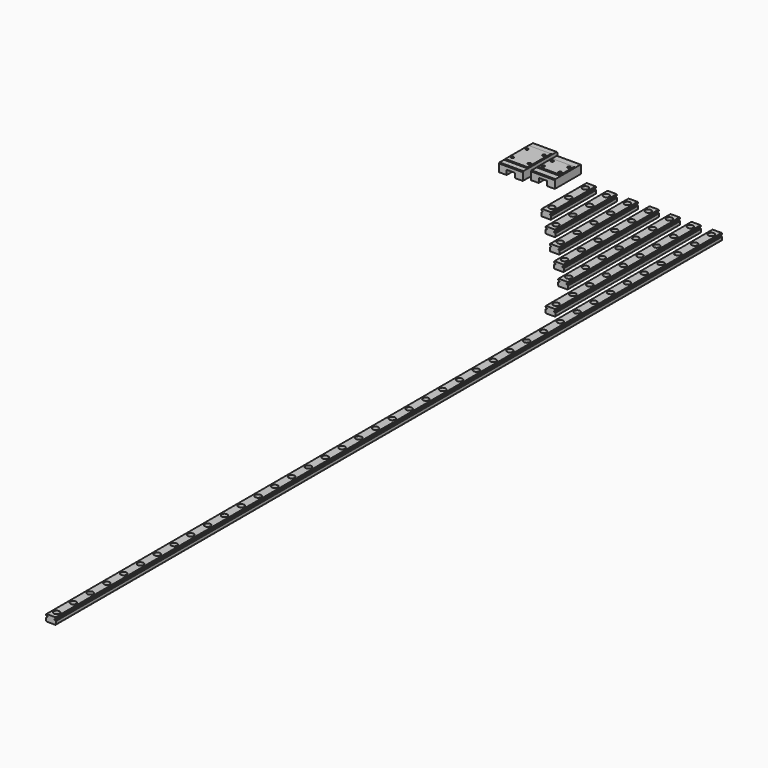
from build123d import *

# Parameters (mm, degrees)
F1_DEPTH         = 40
F2_DEPTH         = 55
F3_DEPTH         = 70
F4_DEPTH         = 85
F5_DEPTH         = 100
F6_DEPTH         = 130
F7_DEPTH         = 595
F9_D             = 2.4
F9_CBORE_D       = 4.2
F9_CBORE_DEPTH   = 2.3
F9_2_D           = 2.4
F9_2_CBORE_D     = 4.2
F9_2_CBORE_DEPTH = 2.3
F9_3_D           = 2.4
F9_3_CBORE_D     = 4.2
F9_3_CBORE_DEPTH = 2.3
F9_4_D           = 2.4
F9_4_CBORE_D     = 4.2
F9_4_CBORE_DEPTH = 2.3
F9_5_D           = 2.4
F9_5_CBORE_D     = 4.2
F9_5_CBORE_DEPTH = 2.3
F9_6_D           = 2.4
F9_6_CBORE_D     = 4.2
F9_6_CBORE_DEPTH = 2.3
F9_7_D           = 2.4
F9_7_CBORE_D     = 4.2
F9_7_CBORE_DEPTH = 2.3
F11_DEPTH        = 6.75
F13_DEPTH        = 5
F14_DEPTH        = 10.9
F16_DEPTH        = 4.5
F18_D            = 2
F18_DEPTH        = 2.5
F18_TIP          = 0.600860619
F18_2_D          = 2
F18_2_DEPTH      = 2.5
F18_2_TIP        = 0.600860619
F19_SIZE         = 0.49999
F19_2_SIZE       = 0.49999


# Not quite as in the source:
# - a fillet or chamfer is up to 0.001 mm smaller than in the source, because OpenCascade refuses the exact size


with BuildPart() as f1:
    # F0 (on Front) → F1 (new body)
    with BuildSketch(Plane.XZ):
        with BuildLine():
            Line((-3.2171572875, -2.4), (3.2171572875, -2.4))
            Line((3.2171572875, -2.4), (3.5, -2.1171572875))
            Line((3.5, -2.1171572875), (3.5, 0.1030976998))
            ThreePointArc((3.5, 0.1030976998), (3.2252249424, 0.2606627579), (3.036437636, 0.515))
            Line((3.036437636, 0.515), (2.6, 0.515))
            Line((2.6, 0.515), (2.6, 1.165))
            Line((2.6, 1.165), (3.036437636, 1.165))
            ThreePointArc((3.036437636, 1.165), (3.2252249424, 1.4193372421), (3.5, 1.5769023002))
            Line((3.5, 1.5769023002), (3.5, 2.1171572875))
            Line((3.5, 2.1171572875), (3.2171572875, 2.4))
            Line((3.2171572875, 2.4), (-3.2171572875, 2.4))
            Line((-3.2171572875, 2.4), (-3.5, 2.1171572875))
            Line((-3.5, 2.1171572875), (-3.5, 1.5769023002))
            ThreePointArc((-3.5, 1.5769023002), (-3.2252249424, 1.4193372421), (-3.036437636, 1.165))
            Line((-3.036437636, 1.165), (-2.6, 1.165))
            Line((-2.6, 1.165), (-2.6, 0.515))
            Line((-2.6, 0.515), (-3.036437636, 0.515))
            ThreePointArc((-3.036437636, 0.515), (-3.2252249424, 0.2606627579), (-3.5, 0.1030976998))
            Line((-3.5, 0.1030976998), (-3.5, -2.1171572875))
            Line((-3.5, -2.1171572875), (-3.2171572875, -2.4))
        make_face()
    extrude(amount=F1_DEPTH)

    # F9 (through all)
    with Locations(Plane.XY.offset(2.4)):
        with Locations((0, -5), (0, -20), (0, -35), (15, -5), (15, -20), (15, -35), (15, -50), (30, -5), (45, -5), (60, -5), (75, -5), (90, -5), (60, -20), (45, -20), (30, -20), (60, -35), (90, -65), (90, -50), (45, -50), (45, -35), (75, -50), (75, -65), (30, -50), (30, -35), (60, -65), (60, -50), (45, -65), (30, -65), (90, -35), (90, -20), (75, -20), (75, -35), (90, -95), (75, -95), (60, -95), (90, -110), (75, -110), (90, -125), (75, -125), (90, -80), (75, -80), (60, -80), (45, -80), (90, -305), (90, -290), (90, -215), (90, -200), (90, -185), (90, -350), (90, -320), (90, -335), (90, -245), (90, -230), (90, -140), (90, -365), (90, -380), (90, -260), (90, -275), (90, -395), (90, -155), (90, -170), (90, -530), (90, -545), (90, -455), (90, -440), (90, -425), (90, -560), (90, -575), (90, -590), (90, -470), (90, -485), (90, -500), (90, -515), (90, -410), (90, -410), (90, -425), (90, -440), (90, -455), (90, -470), (90, -485), (90, -500), (90, -515), (90, -530), (90, -545), (90, -560), (90, -575), (90, -590)):
            CounterBoreHole(F9_D / 2, F9_CBORE_D / 2, F9_CBORE_DEPTH)


with BuildPart() as f2:
    # F0 (on Front) → F2 (new body)
    with BuildSketch(Plane.XZ):
        with BuildLine():
            Line((11.5, 0.1030976998), (11.5, -2.1171572875))
            Line((11.5, -2.1171572875), (11.7828427125, -2.4))
            Line((11.7828427125, -2.4), (18.2171572875, -2.4))
            Line((18.2171572875, -2.4), (18.5, -2.1171572875))
            Line((18.5, -2.1171572875), (18.5, 0.1030976998))
            ThreePointArc((18.5, 0.1030976998), (18.2252249424, 0.2606627579), (18.036437636, 0.515))
            Line((18.036437636, 0.515), (17.6, 0.515))
            Line((17.6, 0.515), (17.6, 1.165))
            Line((17.6, 1.165), (18.036437636, 1.165))
            ThreePointArc((18.036437636, 1.165), (18.2252249424, 1.4193372421), (18.5, 1.5769023002))
            Line((18.5, 1.5769023002), (18.5, 2.1171572875))
            Line((18.5, 2.1171572875), (18.2171572875, 2.4))
            Line((18.2171572875, 2.4), (11.7828427125, 2.4))
            Line((11.7828427125, 2.4), (11.5, 2.1171572875))
            Line((11.5, 2.1171572875), (11.5, 1.5769023002))
            ThreePointArc((11.5, 1.5769023002), (11.7747750576, 1.4193372421), (11.963562364, 1.165))
            Line((11.963562364, 1.165), (12.4, 1.165))
            Line((12.4, 1.165), (12.4, 0.515))
            Line((12.4, 0.515), (11.963562364, 0.515))
            ThreePointArc((11.963562364, 0.515), (11.7747750576, 0.2606627579), (11.5, 0.1030976998))
        make_face()
    extrude(amount=F2_DEPTH)

    # F9#2 (through all)
    with Locations(Plane.XY.offset(2.4)):
        with Locations((0, -5), (0, -20), (0, -35), (15, -5), (15, -20), (15, -35), (15, -50), (30, -5), (45, -5), (60, -5), (75, -5), (90, -5), (60, -20), (45, -20), (30, -20), (60, -35), (90, -65), (90, -50), (45, -50), (45, -35), (75, -50), (75, -65), (30, -50), (30, -35), (60, -65), (60, -50), (45, -65), (30, -65), (90, -35), (90, -20), (75, -20), (75, -35), (90, -95), (75, -95), (60, -95), (90, -110), (75, -110), (90, -125), (75, -125), (90, -80), (75, -80), (60, -80), (45, -80), (90, -305), (90, -290), (90, -215), (90, -200), (90, -185), (90, -350), (90, -320), (90, -335), (90, -245), (90, -230), (90, -140), (90, -365), (90, -380), (90, -260), (90, -275), (90, -395), (90, -155), (90, -170), (90, -530), (90, -545), (90, -455), (90, -440), (90, -425), (90, -560), (90, -575), (90, -590), (90, -470), (90, -485), (90, -500), (90, -515), (90, -410), (90, -410), (90, -425), (90, -440), (90, -455), (90, -470), (90, -485), (90, -500), (90, -515), (90, -530), (90, -545), (90, -560), (90, -575), (90, -590)):
            CounterBoreHole(F9_2_D / 2, F9_2_CBORE_D / 2, F9_2_CBORE_DEPTH)


with BuildPart() as f3:
    # F0 (on Front) → F3 (new body)
    with BuildSketch(Plane.XZ):
        with BuildLine():
            Line((26.5, 0.1030976998), (26.5, -2.1171572875))
            Line((26.5, -2.1171572875), (26.7828427125, -2.4))
            Line((26.7828427125, -2.4), (33.2171572875, -2.4))
            Line((33.2171572875, -2.4), (33.5, -2.1171572875))
            Line((33.5, -2.1171572875), (33.5, 0.1030976998))
            ThreePointArc((33.5, 0.1030976998), (33.2252249424, 0.2606627579), (33.036437636, 0.515))
            Line((33.036437636, 0.515), (32.6, 0.515))
            Line((32.6, 0.515), (32.6, 1.165))
            Line((32.6, 1.165), (33.036437636, 1.165))
            ThreePointArc((33.036437636, 1.165), (33.2252249424, 1.4193372421), (33.5, 1.5769023002))
            Line((33.5, 1.5769023002), (33.5, 2.1171572875))
            Line((33.5, 2.1171572875), (33.2171572875, 2.4))
            Line((33.2171572875, 2.4), (26.7828427125, 2.4))
            Line((26.7828427125, 2.4), (26.5, 2.1171572875))
            Line((26.5, 2.1171572875), (26.5, 1.5769023002))
            ThreePointArc((26.5, 1.5769023002), (26.7747750576, 1.4193372421), (26.963562364, 1.165))
            Line((26.963562364, 1.165), (27.4, 1.165))
            Line((27.4, 1.165), (27.4, 0.515))
            Line((27.4, 0.515), (26.963562364, 0.515))
            ThreePointArc((26.963562364, 0.515), (26.7747750576, 0.2606627579), (26.5, 0.1030976998))
        make_face()
    extrude(amount=F3_DEPTH)

    # F9#3 (through all)
    with Locations(Plane.XY.offset(2.4)):
        with Locations((0, -5), (0, -20), (0, -35), (15, -5), (15, -20), (15, -35), (15, -50), (30, -5), (45, -5), (60, -5), (75, -5), (90, -5), (60, -20), (45, -20), (30, -20), (60, -35), (90, -65), (90, -50), (45, -50), (45, -35), (75, -50), (75, -65), (30, -50), (30, -35), (60, -65), (60, -50), (45, -65), (30, -65), (90, -35), (90, -20), (75, -20), (75, -35), (90, -95), (75, -95), (60, -95), (90, -110), (75, -110), (90, -125), (75, -125), (90, -80), (75, -80), (60, -80), (45, -80), (90, -305), (90, -290), (90, -215), (90, -200), (90, -185), (90, -350), (90, -320), (90, -335), (90, -245), (90, -230), (90, -140), (90, -365), (90, -380), (90, -260), (90, -275), (90, -395), (90, -155), (90, -170), (90, -530), (90, -545), (90, -455), (90, -440), (90, -425), (90, -560), (90, -575), (90, -590), (90, -470), (90, -485), (90, -500), (90, -515), (90, -410), (90, -410), (90, -425), (90, -440), (90, -455), (90, -470), (90, -485), (90, -500), (90, -515), (90, -530), (90, -545), (90, -560), (90, -575), (90, -590)):
            CounterBoreHole(F9_3_D / 2, F9_3_CBORE_D / 2, F9_3_CBORE_DEPTH)


with BuildPart() as f4:
    # F0 (on Front) → F4 (new body)
    with BuildSketch(Plane.XZ):
        with BuildLine():
            Line((41.5, 0.1030976998), (41.5, -2.1171572875))
            Line((41.5, -2.1171572875), (41.7828427125, -2.4))
            Line((41.7828427125, -2.4), (48.2171572875, -2.4))
            Line((48.2171572875, -2.4), (48.5, -2.1171572875))
            Line((48.5, -2.1171572875), (48.5, 0.1030976998))
            ThreePointArc((48.5, 0.1030976998), (48.2252249424, 0.2606627579), (48.036437636, 0.515))
            Line((48.036437636, 0.515), (47.6, 0.515))
            Line((47.6, 0.515), (47.6, 1.165))
            Line((47.6, 1.165), (48.036437636, 1.165))
            ThreePointArc((48.036437636, 1.165), (48.2252249424, 1.4193372421), (48.5, 1.5769023002))
            Line((48.5, 1.5769023002), (48.5, 2.1171572875))
            Line((48.5, 2.1171572875), (48.2171572875, 2.4))
            Line((48.2171572875, 2.4), (41.7828427125, 2.4))
            Line((41.7828427125, 2.4), (41.5, 2.1171572875))
            Line((41.5, 2.1171572875), (41.5, 1.5769023002))
            ThreePointArc((41.5, 1.5769023002), (41.7747750576, 1.4193372421), (41.963562364, 1.165))
            Line((41.963562364, 1.165), (42.4, 1.165))
            Line((42.4, 1.165), (42.4, 0.515))
            Line((42.4, 0.515), (41.963562364, 0.515))
            ThreePointArc((41.963562364, 0.515), (41.7747750576, 0.2606627579), (41.5, 0.1030976998))
        make_face()
    extrude(amount=F4_DEPTH)

    # F9#4 (through all)
    with Locations(Plane.XY.offset(2.4)):
        with Locations((0, -5), (0, -20), (0, -35), (15, -5), (15, -20), (15, -35), (15, -50), (30, -5), (45, -5), (60, -5), (75, -5), (90, -5), (60, -20), (45, -20), (30, -20), (60, -35), (90, -65), (90, -50), (45, -50), (45, -35), (75, -50), (75, -65), (30, -50), (30, -35), (60, -65), (60, -50), (45, -65), (30, -65), (90, -35), (90, -20), (75, -20), (75, -35), (90, -95), (75, -95), (60, -95), (90, -110), (75, -110), (90, -125), (75, -125), (90, -80), (75, -80), (60, -80), (45, -80), (90, -305), (90, -290), (90, -215), (90, -200), (90, -185), (90, -350), (90, -320), (90, -335), (90, -245), (90, -230), (90, -140), (90, -365), (90, -380), (90, -260), (90, -275), (90, -395), (90, -155), (90, -170), (90, -530), (90, -545), (90, -455), (90, -440), (90, -425), (90, -560), (90, -575), (90, -590), (90, -470), (90, -485), (90, -500), (90, -515), (90, -410), (90, -410), (90, -425), (90, -440), (90, -455), (90, -470), (90, -485), (90, -500), (90, -515), (90, -530), (90, -545), (90, -560), (90, -575), (90, -590)):
            CounterBoreHole(F9_4_D / 2, F9_4_CBORE_D / 2, F9_4_CBORE_DEPTH)


with BuildPart() as f5:
    # F0 (on Front) → F5 (new body)
    with BuildSketch(Plane.XZ):
        with BuildLine():
            Line((56.5, 0.1030976998), (56.5, -2.1171572875))
            Line((56.5, -2.1171572875), (56.7828427125, -2.4))
            Line((56.7828427125, -2.4), (63.2171572875, -2.4))
            Line((63.2171572875, -2.4), (63.5, -2.1171572875))
            Line((63.5, -2.1171572875), (63.5, 0.1030976998))
            ThreePointArc((63.5, 0.1030976998), (63.2252249424, 0.2606627579), (63.036437636, 0.515))
            Line((63.036437636, 0.515), (62.6, 0.515))
            Line((62.6, 0.515), (62.6, 1.165))
            Line((62.6, 1.165), (63.036437636, 1.165))
            ThreePointArc((63.036437636, 1.165), (63.2252249424, 1.4193372421), (63.5, 1.5769023002))
            Line((63.5, 1.5769023002), (63.5, 2.1171572875))
            Line((63.5, 2.1171572875), (63.2171572875, 2.4))
            Line((63.2171572875, 2.4), (56.7828427125, 2.4))
            Line((56.7828427125, 2.4), (56.5, 2.1171572875))
            Line((56.5, 2.1171572875), (56.5, 1.5769023002))
            ThreePointArc((56.5, 1.5769023002), (56.7747750576, 1.4193372421), (56.963562364, 1.165))
            Line((56.963562364, 1.165), (57.4, 1.165))
            Line((57.4, 1.165), (57.4, 0.515))
            Line((57.4, 0.515), (56.963562364, 0.515))
            ThreePointArc((56.963562364, 0.515), (56.7747750576, 0.2606627579), (56.5, 0.1030976998))
        make_face()
    extrude(amount=F5_DEPTH)

    # F9#5 (through all)
    with Locations(Plane.XY.offset(2.4)):
        with Locations((0, -5), (0, -20), (0, -35), (15, -5), (15, -20), (15, -35), (15, -50), (30, -5), (45, -5), (60, -5), (75, -5), (90, -5), (60, -20), (45, -20), (30, -20), (60, -35), (90, -65), (90, -50), (45, -50), (45, -35), (75, -50), (75, -65), (30, -50), (30, -35), (60, -65), (60, -50), (45, -65), (30, -65), (90, -35), (90, -20), (75, -20), (75, -35), (90, -95), (75, -95), (60, -95), (90, -110), (75, -110), (90, -125), (75, -125), (90, -80), (75, -80), (60, -80), (45, -80), (90, -305), (90, -290), (90, -215), (90, -200), (90, -185), (90, -350), (90, -320), (90, -335), (90, -245), (90, -230), (90, -140), (90, -365), (90, -380), (90, -260), (90, -275), (90, -395), (90, -155), (90, -170), (90, -530), (90, -545), (90, -455), (90, -440), (90, -425), (90, -560), (90, -575), (90, -590), (90, -470), (90, -485), (90, -500), (90, -515), (90, -410), (90, -410), (90, -425), (90, -440), (90, -455), (90, -470), (90, -485), (90, -500), (90, -515), (90, -530), (90, -545), (90, -560), (90, -575), (90, -590)):
            CounterBoreHole(F9_5_D / 2, F9_5_CBORE_D / 2, F9_5_CBORE_DEPTH)


with BuildPart() as f6:
    # F0 (on Front) → F6 (new body)
    with BuildSketch(Plane.XZ):
        with BuildLine():
            Line((71.5, 0.1030976998), (71.5, -2.1171572875))
            Line((71.5, -2.1171572875), (71.7828427125, -2.4))
            Line((71.7828427125, -2.4), (78.2171572875, -2.4))
            Line((78.2171572875, -2.4), (78.5, -2.1171572875))
            Line((78.5, -2.1171572875), (78.5, 0.1030976998))
            ThreePointArc((78.5, 0.1030976998), (78.2252249424, 0.2606627579), (78.036437636, 0.515))
            Line((78.036437636, 0.515), (77.6, 0.515))
            Line((77.6, 0.515), (77.6, 1.165))
            Line((77.6, 1.165), (78.036437636, 1.165))
            ThreePointArc((78.036437636, 1.165), (78.2252249424, 1.4193372421), (78.5, 1.5769023002))
            Line((78.5, 1.5769023002), (78.5, 2.1171572875))
            Line((78.5, 2.1171572875), (78.2171572875, 2.4))
            Line((78.2171572875, 2.4), (71.7828427125, 2.4))
            Line((71.7828427125, 2.4), (71.5, 2.1171572875))
            Line((71.5, 2.1171572875), (71.5, 1.5769023002))
            ThreePointArc((71.5, 1.5769023002), (71.7747750576, 1.4193372421), (71.963562364, 1.165))
            Line((71.963562364, 1.165), (72.4, 1.165))
            Line((72.4, 1.165), (72.4, 0.515))
            Line((72.4, 0.515), (71.963562364, 0.515))
            ThreePointArc((71.963562364, 0.515), (71.7747750576, 0.2606627579), (71.5, 0.1030976998))
        make_face()
    extrude(amount=F6_DEPTH)

    # F9#6 (through all)
    with Locations(Plane.XY.offset(2.4)):
        with Locations((0, -5), (0, -20), (0, -35), (15, -5), (15, -20), (15, -35), (15, -50), (30, -5), (45, -5), (60, -5), (75, -5), (90, -5), (60, -20), (45, -20), (30, -20), (60, -35), (90, -65), (90, -50), (45, -50), (45, -35), (75, -50), (75, -65), (30, -50), (30, -35), (60, -65), (60, -50), (45, -65), (30, -65), (90, -35), (90, -20), (75, -20), (75, -35), (90, -95), (75, -95), (60, -95), (90, -110), (75, -110), (90, -125), (75, -125), (90, -80), (75, -80), (60, -80), (45, -80), (90, -305), (90, -290), (90, -215), (90, -200), (90, -185), (90, -350), (90, -320), (90, -335), (90, -245), (90, -230), (90, -140), (90, -365), (90, -380), (90, -260), (90, -275), (90, -395), (90, -155), (90, -170), (90, -530), (90, -545), (90, -455), (90, -440), (90, -425), (90, -560), (90, -575), (90, -590), (90, -470), (90, -485), (90, -500), (90, -515), (90, -410), (90, -410), (90, -425), (90, -440), (90, -455), (90, -470), (90, -485), (90, -500), (90, -515), (90, -530), (90, -545), (90, -560), (90, -575), (90, -590)):
            CounterBoreHole(F9_6_D / 2, F9_6_CBORE_D / 2, F9_6_CBORE_DEPTH)


with BuildPart() as f7:
    # F0 (on Front) → F7 (new body)
    with BuildSketch(Plane.XZ):
        with BuildLine():
            Line((86.5, 0.1030976998), (86.5, -2.1171572875))
            Line((86.5, -2.1171572875), (86.7828427125, -2.4))
            Line((86.7828427125, -2.4), (93.2171572875, -2.4))
            Line((93.2171572875, -2.4), (93.5, -2.1171572875))
            Line((93.5, -2.1171572875), (93.5, 0.1030976998))
            ThreePointArc((93.5, 0.1030976998), (93.2252249424, 0.2606627579), (93.036437636, 0.515))
            Line((93.036437636, 0.515), (92.6, 0.515))
            Line((92.6, 0.515), (92.6, 1.165))
            Line((92.6, 1.165), (93.036437636, 1.165))
            ThreePointArc((93.036437636, 1.165), (93.2252249424, 1.4193372421), (93.5, 1.5769023002))
            Line((93.5, 1.5769023002), (93.5, 2.1171572875))
            Line((93.5, 2.1171572875), (93.2171572875, 2.4))
            Line((93.2171572875, 2.4), (86.7828427125, 2.4))
            Line((86.7828427125, 2.4), (86.5, 2.1171572875))
            Line((86.5, 2.1171572875), (86.5, 1.5769023002))
            ThreePointArc((86.5, 1.5769023002), (86.7747750576, 1.4193372421), (86.963562364, 1.165))
            Line((86.963562364, 1.165), (87.4, 1.165))
            Line((87.4, 1.165), (87.4, 0.515))
            Line((87.4, 0.515), (86.963562364, 0.515))
            ThreePointArc((86.963562364, 0.515), (86.7747750576, 0.2606627579), (86.5, 0.1030976998))
        make_face()
    extrude(amount=F7_DEPTH)

    # F9#7 (through all)
    with Locations(Plane.XY.offset(2.4)):
        with Locations((0, -5), (0, -20), (0, -35), (15, -5), (15, -20), (15, -35), (15, -50), (30, -5), (45, -5), (60, -5), (75, -5), (90, -5), (60, -20), (45, -20), (30, -20), (60, -35), (90, -65), (90, -50), (45, -50), (45, -35), (75, -50), (75, -65), (30, -50), (30, -35), (60, -65), (60, -50), (45, -65), (30, -65), (90, -35), (90, -20), (75, -20), (75, -35), (90, -95), (75, -95), (60, -95), (90, -110), (75, -110), (90, -125), (75, -125), (90, -80), (75, -80), (60, -80), (45, -80), (90, -305), (90, -290), (90, -215), (90, -200), (90, -185), (90, -350), (90, -320), (90, -335), (90, -245), (90, -230), (90, -140), (90, -365), (90, -380), (90, -260), (90, -275), (90, -395), (90, -155), (90, -170), (90, -530), (90, -545), (90, -455), (90, -440), (90, -425), (90, -560), (90, -575), (90, -590), (90, -470), (90, -485), (90, -500), (90, -515), (90, -410), (90, -410), (90, -425), (90, -440), (90, -455), (90, -470), (90, -485), (90, -500), (90, -515), (90, -530), (90, -545), (90, -560), (90, -575), (90, -590)):
            CounterBoreHole(F9_7_D / 2, F9_7_CBORE_D / 2, F9_7_CBORE_DEPTH)


with BuildPart() as f11:
    # F10 (on Front) → F11 (new body)
    with BuildSketch(Plane.XZ):
        with BuildLine():
            Line((-16.5, 5.1), (-33.5, 5.1))
            Line((-33.5, 5.1), (-33.5, -0.9))
            Line((-33.5, -0.9), (-28, -0.9))
            Line((-28, -0.9), (-28, 0.065))
            ThreePointArc((-28, 0.065), (-28.775, 0.84), (-28, 1.615))
            Line((-28, 1.615), (-28, 2.4))
            Line((-28, 2.4), (-25, 2.4))
            Line((-25, 2.4), (-22, 2.4))
            Line((-22, 2.4), (-22, 1.615))
            ThreePointArc((-22, 1.615), (-21.225, 0.84), (-22, 0.065))
            Line((-22, 0.065), (-22, -0.9))
            Line((-22, -0.9), (-16.5, -0.9))
            Line((-16.5, -0.9), (-16.5, 5.1))
        make_face()
        Polygon((-16.5, 5.6), (-25, 5.6), (-33.5, 5.6), (-33.5, 5.1), (-16.5, 5.1), align=None)
    extrude(amount=F11_DEPTH)

    # F12 (on face) → F13 (join)
    with BuildSketch(Plane.XZ.offset(6.75)):
        with BuildLine():
            Line((-28, -0.9), (-28, 0.065))
            ThreePointArc((-28, 0.065), (-28.775, 0.84), (-28, 1.615))
            Line((-28, 1.615), (-28, 2.4))
            Line((-28, 2.4), (-22, 2.4))
            Line((-22, 2.4), (-22, 1.615))
            ThreePointArc((-22, 1.615), (-21.225, 0.84), (-22, 0.065))
            Line((-22, 0.065), (-22, -0.9))
            Line((-22, -0.9), (-16.5, -0.9))
            Line((-16.5, -0.9), (-16.5, 5.1))
            Line((-16.5, 5.1), (-33.5, 5.1))
            Line((-33.5, 5.1), (-33.5, -0.9))
            Line((-33.5, -0.9), (-28, -0.9))
        make_face()
        with BuildLine():
            ThreePointArc((-28, 1.615), (-28.775, 0.84), (-28, 0.065))
            Line((-28, 0.065), (-28, 1.615))
        make_face()
        with BuildLine():
            ThreePointArc((-22, 0.065), (-21.225, 0.84), (-22, 1.615))
            Line((-22, 1.615), (-22, 0.065))
        make_face()
    extrude(amount=F13_DEPTH)

    # F18
    with Locations(Plane.XY.offset(5.6)):
        with Locations((-31, -4), (-19, -4), (-39, -6.5), (-51, -6.5)):
            Hole(F18_D / 2, depth=F18_DEPTH)
            with Locations((0, 0, -(F18_DEPTH + F18_TIP / 2))):  # 118° drill point
                Cone(0, F18_D / 2, F18_TIP, mode=Mode.SUBTRACT)

    # F19 (size 0.5 in the source; OpenCascade refuses exactly that, so slightly less here)
    f19_edges = [f11.edges().sort_by_distance(p)[0] for p in [
        (-25, -6.75, 5.6),
        (-16.5, -3.375, 5.6),
        (-25, -11.75, 5.1),
        (-33.5, -3.375, 5.6),
    ]]
    chamfer(f19_edges, length=F19_SIZE)



with BuildPart() as f14:
    # F10 (on Front) → F14 (new body)
    with BuildSketch(Plane.XZ):
        with BuildLine():
            Line((-53.5, -0.9), (-48, -0.9))
            Line((-48, -0.9), (-48, 0.065))
            ThreePointArc((-48, 0.065), (-48.775, 0.84), (-48, 1.615))
            Line((-48, 1.615), (-48, 2.4))
            Line((-48, 2.4), (-45, 2.4))
            Line((-45, 2.4), (-42, 2.4))
            Line((-42, 2.4), (-42, 1.615))
            ThreePointArc((-42, 1.615), (-41.225, 0.84), (-42, 0.065))
            Line((-42, 0.065), (-42, -0.9))
            Line((-42, -0.9), (-36.5, -0.9))
            Line((-36.5, -0.9), (-36.5, 5.1))
            Line((-36.5, 5.1), (-53.5, 5.1))
            Line((-53.5, 5.1), (-53.5, -0.9))
        make_face()
        Polygon((-53.5, 5.6), (-53.5, 5.1), (-36.5, 5.1), (-36.5, 5.6), (-45, 5.6), align=None)
    extrude(amount=F14_DEPTH)

    # F15 (on face) → F16 (join)
    with BuildSketch(Plane.XZ.offset(10.9)):
        with BuildLine():
            Line((-48, -0.9), (-48, 0.065))
            ThreePointArc((-48, 0.065), (-48.775, 0.84), (-48, 1.615))
            Line((-48, 1.615), (-48, 2.4))
            Line((-48, 2.4), (-42, 2.4))
            Line((-42, 2.4), (-42, 1.615))
            ThreePointArc((-42, 1.615), (-41.225, 0.84), (-42, 0.065))
            Line((-42, 0.065), (-42, -0.9))
            Line((-42, -0.9), (-36.5, -0.9))
            Line((-36.5, -0.9), (-36.5, 5.1))
            Line((-36.5, 5.1), (-53.5, 5.1))
            Line((-53.5, 5.1), (-53.5, -0.9))
            Line((-53.5, -0.9), (-48, -0.9))
        make_face()
        with BuildLine():
            ThreePointArc((-48, 1.615), (-48.775, 0.84), (-48, 0.065))
            Line((-48, 0.065), (-48, 1.615))
        make_face()
        with BuildLine():
            ThreePointArc((-42, 0.065), (-41.225, 0.84), (-42, 1.615))
            Line((-42, 1.615), (-42, 0.065))
        make_face()
    extrude(amount=F16_DEPTH)

    # F18#2
    with Locations(Plane.XY.offset(5.6)):
        with Locations((-31, -4), (-19, -4), (-39, -6.5), (-51, -6.5)):
            Hole(F18_2_D / 2, depth=F18_2_DEPTH)
            with Locations((0, 0, -(F18_2_DEPTH + F18_2_TIP / 2))):  # 118° drill point
                Cone(0, F18_2_D / 2, F18_2_TIP, mode=Mode.SUBTRACT)

    # F19#2 (size 0.5 in the source; OpenCascade refuses exactly that, so slightly less here)
    f19_2_edges = [f14.edges().sort_by_distance(p)[0] for p in [
        (-45, -15.4, 5.1),
        (-45, -10.9, 5.6),
        (-36.5, -5.45, 5.6),
        (-53.5, -5.45, 5.6),
    ]]
    chamfer(f19_2_edges, length=F19_2_SIZE)


with BuildPart() as f11_1:
    add(f11.part)

    add(f14.part)  # F20 merges F14
    # F20: F14, F11 across face
    add(f14.part.mirror(Plane(origin=(-25, 0, 2.7311796104), x_dir=(1, 0, 0), z_dir=(0, 1, 0))))
    add(f11.part.mirror(Plane(origin=(-25, 0, 2.7311796104), x_dir=(1, 0, 0), z_dir=(0, 1, 0))))


solid = Compound([f1.part, f2.part, f3.part, f4.part, f5.part, f6.part, f7.part, f11_1.part])
